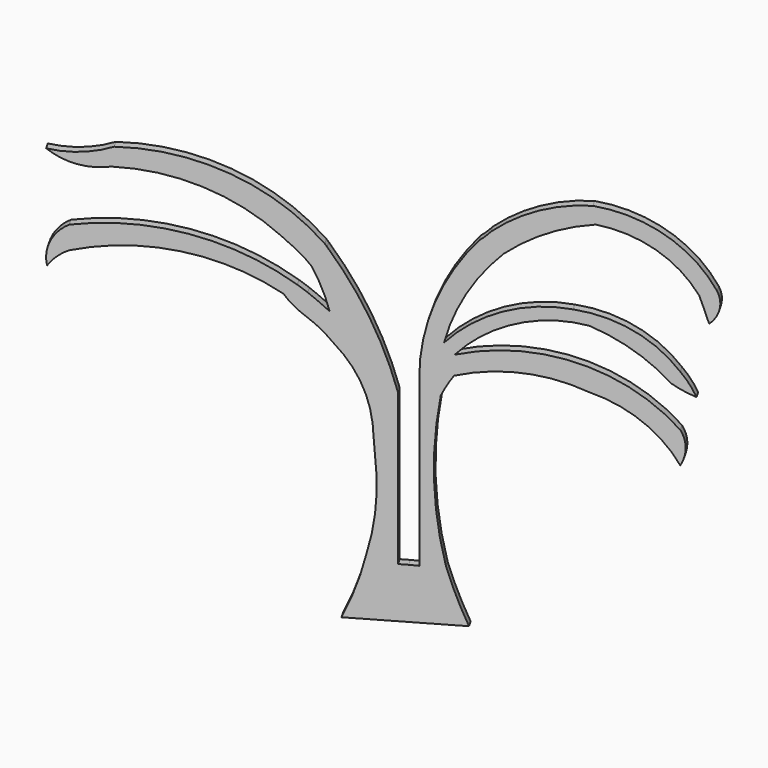
from build123d import *

# Parameters (mm, degrees)
F1_DEPTH = 25.4
F2_ANGLE = 240
F3_ANGLE = 30


# Not quite as in the source:
# - a feature names something its author has since deleted; it is built from what else it names


with BuildPart() as f1:
    # F0 (on Front) → F1 (new body)
    with BuildSketch(Plane.XZ):
        with BuildLine():
            ThreePointArc((250.1826790571, 167.252155113), (278.1130880831, 191.8897284489), (301.4146556953, 220.9440691755))
            ThreePointArc((301.4146556953, 220.9440691755), (548.9344062192, 315.2980350064), (813.1931424143, 296.9672381879))
            ThreePointArc((813.1931424143, 296.9672381879), (843.2368199295, 278.4857074323), (866.6267395021, 252.0830333234))
            ThreePointArc((866.6267395021, 252.0830333234), (859.2886133314, 317.8635284318), (813.1931424141, 365.3622567654))
            ThreePointArc((813.1931424141, 365.3622567654), (528.658381188, 363.1008503302), (268.4933890423, 247.8649133709))
            ThreePointArc((268.4933890423, 247.8649133709), (255.8828799715, 238.6195077853), (243.4818595648, 229.0949523449))
            ThreePointArc((243.4818595648, 229.0949523449), (216.8466348082, 206.3937348312), (191.0419305212, 182.7527172748))
            ThreePointArc((191.0419305212, 182.7527172748), (209.2426753746, 242.3856524278), (234.085008502, 299.5714247227))
            ThreePointArc((234.085008502, 299.5714247227), (262.5639500876, 333.6377098113), (295.1646447182, 363.7832999229))
            ThreePointArc((295.1646447182, 363.7832999229), (301.1050415282, 369.5098935095), (307.1268496022, 375.1508168282))
            ThreePointArc((307.1268496022, 375.1508168282), (495.0303186662, 491.0726231916), (712.7380371094, 527.8003811836))
            ThreePointArc((712.7380371094, 527.8003811836), (794.9345928524, 528.0032351591), (868.764102459, 564.1351938248))
            ThreePointArc((868.764102459, 564.1351938248), (786.3289991041, 561.1323579191), (706.3259482384, 581.2339782715))
            ThreePointArc((706.3259482384, 581.2339782715), (428.7633374116, 531.0006025963), (202.7621120214, 362.2171878815))
            ThreePointArc((202.7621120214, 362.2171878815), (199.8950650536, 358.0887688295), (197.0456982791, 353.9481274337))
            ThreePointArc((197.0456982791, 353.9481274337), (95.8778868485, 174.2465451031), (27.6736820157, -20.3704408073))
            Line((27.6736820157, -20.3704408073), (27.6736820157, -477.5704408073))
            Line((27.6736820157, -477.5704408073), (2.2736820157, -477.5704408073))
            Line((2.2736820157, -477.5704408073), (-23.1156889348, -478.3051807189))
            Line((-23.1156889348, -478.3051807189), (-23.1156889348, -20.3704408073))
            Line((-23.1156889348, -20.3704408073), (-23.1156889348, 23.7159409966))
            ThreePointArc((-23.1156889348, 23.7159409966), (-60.1684665025, 225.1338478784), (-166.475340724, 400.1793563366))
            ThreePointArc((-166.475340724, 400.1793563366), (-181.4907758471, 412.3365760313), (-195.1139737362, 426.0358373953))
            ThreePointArc((-195.1139737362, 426.0358373953), (-309.3402704075, 490.6134334), (-438.5659396648, 513.3870840073))
            ThreePointArc((-438.5659396648, 513.3870840073), (-612.4676441027, 448.3168030455), (-735.3243231773, 309.0969026089))
            ThreePointArc((-735.3243231773, 309.0969026089), (-741.1111301221, 261.6187426822), (-715.9704566002, 220.9295630455))
            ThreePointArc((-715.9704566002, 220.9295630455), (-704.4880158315, 257.5983242076), (-692.3158168793, 294.0439283848))
            ThreePointArc((-692.3158168793, 294.0439283848), (-588.6352200974, 408.0539998704), (-445.0172185898, 463.9273583889))
            ThreePointArc((-445.0172185898, 463.9273583889), (-328.3620257934, 431.1988717022), (-224.5548516512, 368.7196075916))
            ThreePointArc((-224.5548516512, 368.7196075916), (-135.4578046593, 255.1906523593), (-82.276083529, 121.0310012102))
            ThreePointArc((-82.276083529, 121.0310012102), (-222.8986090653, 214.7399937609), (-390.8064365387, 233.7933778763))
            ThreePointArc((-390.8064365387, 233.7933778763), (-534.8506307826, 188.5252288055), (-647.1569538116, 87.6033529639))
            ThreePointArc((-647.1569538116, 87.6033529639), (-668.750342933, 56.6907627964), (-685.8645677567, 23.0906736106))
            ThreePointArc((-685.8645677567, 23.0906736106), (-654.782784529, 37.0530177531), (-625.6527304649, 54.7296761702))
            ThreePointArc((-625.6527304649, 54.7296761702), (-535.9364621749, 135.4019490396), (-429.9600422382, 193.0736303329))
            ThreePointArc((-429.9600422382, 193.0736303329), (-255.1353162114, 185.0540353391), (-107.6677426965, 90.8133143325))
            ThreePointArc((-107.6677426965, 90.8133143325), (-400.8973120765, 91.9617638291), (-647.1569538116, -67.2270804644))
            ThreePointArc((-647.1569538116, -67.2270804644), (-660.0470579155, -114.5363822579), (-647.1569538116, -161.8456840515))
            ThreePointArc((-647.1569538116, -161.8456840515), (-555.302299834, -51.3433620353), (-428.5768360003, 16.3965630051))
            ThreePointArc((-428.5768360003, 16.3965630051), (-268.955549485, 54.7296761702), (-106.0306501957, 34.633411211))
            ThreePointArc((-106.0306501957, 34.633411211), (-89.072951708, 7.7811719553), (-74.492260997, -20.4324727833))
            ThreePointArc((-74.492260997, -20.4324727833), (-58.44709094, -248.3192131796), (-87.0539037033, -474.9719523956))
            ThreePointArc((-87.0539037033, -474.9719523956), (-111.9092602944, -553.3883298655), (-141.9875799101, -629.9534113053))
            Line((-141.9875799101, -629.9534113053), (162.8124200899, -629.9534113053))
            ThreePointArc((162.8124200899, -629.9534113053), (127.6888612329, -543.8827728043), (102.7497877256, -454.3290916329))
            ThreePointArc((102.7497877256, -454.3290916329), (82.6750571268, -348.4939128162), (79.3961640974, -240.8215916548))
            ThreePointArc((79.3961640974, -240.8215916548), (80.2077016296, -226.8972481017), (81.3018441543, -212.9922565991))
            Line((81.3018441543, -212.9922565991), (87.0378738701, -129.2269402374))
            ThreePointArc((87.0378738701, -129.2269402374), (87.6414479673, -117.6100786674), (88.6270669795, -106.0193785337))
            ThreePointArc((88.6270669795, -106.0193785337), (118.4644160965, 4.4171939804), (182.0192138426, 99.534446014))
            ThreePointArc((182.0192138426, 99.534446014), (213.7444570986, 135.7653016553), (250.1826790571, 167.252155113))
        make_face()
        with BuildLine():
            ThreePointArc((290.310142009, 214.3317525479), (290.308974312, 214.3316774306), (290.3078066153, 214.3316023092))
            Line((290.3078066153, 214.3316023092), (290.7207294437, 214.3993956711))
            ThreePointArc((290.7207294437, 214.3993956711), (290.5154263752, 214.3656308704), (290.310142009, 214.3317525479))
        make_face(mode=Mode.SUBTRACT)
    extrude(amount=F1_DEPTH)


with BuildPart() as f1_1:
    # F2: moved
    add(f1.part.rotate(Axis((27.6736820157, -25.4, -248.9704408073), (0, 0, 1)), F2_ANGLE))


with BuildPart() as f1_2:
    # F3: moved
    add(f1_1.part.rotate(Axis((75.0654127471, 5.8848854854, -227.2946198611), (0, 0, -1)), F3_ANGLE))


solid = f1_2.part
